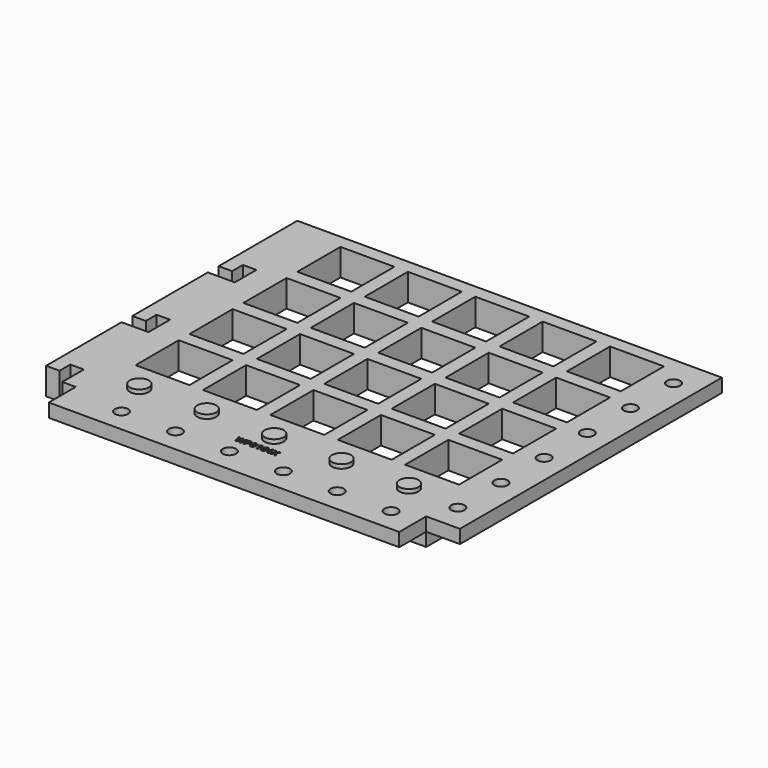
from build123d import *

# Parameters (mm, degrees)
F0_W          = 260
F0_H          = 210
F0_W_2        = 40
F0_H_2        = 40
F1_DEPTH      = 20
F2_DEPTH      = 33
F3_W          = 260
F3_H          = 10
F4_DEPTH      = 25
F5_R          = 4.95
F6_DEPTH      = 25
F7_W          = 243
F7_H          = 10
F8_DEPTH      = 25
F9_R          = 4.95
F10_DEPTH     = 25
F11_W         = 243
F11_H         = 20
F12_DEPTH     = 30
F14_DEPTH     = 25
F15_R         = 7.05
F16_DEPTH     = 3
F17_TEXT_SIZE = 6.9444444444
F18_DEPTH     = 3


# Not quite as in the source:
# - Text() gives the source's letters only with a copy of the font that has no kerning and outlines rounded to 1/6400 em; it was checked with that copy


with BuildPart() as f1:
    # F0 (on Top) → F1 (new body)
    with BuildSketch(Plane.XY):
        Rectangle(F0_W, F0_H)
        with Locations((-100, -75)):
            Rectangle(F0_W_2, F0_H_2, mode=Mode.SUBTRACT)
        with Locations((-50, -75)):
            Rectangle(F0_W_2, F0_H_2, mode=Mode.SUBTRACT)
        with Locations((-100, -25)):
            Rectangle(F0_W_2, F0_H_2, mode=Mode.SUBTRACT)
        with Locations((-50, -25)):
            Rectangle(F0_W_2, F0_H_2, mode=Mode.SUBTRACT)
        with Locations((0, -75)):
            Rectangle(F0_W_2, F0_H_2, mode=Mode.SUBTRACT)
        with Locations((50, -75)):
            Rectangle(F0_W_2, F0_H_2, mode=Mode.SUBTRACT)
        with Locations((100, -75)):
            Rectangle(F0_W_2, F0_H_2, mode=Mode.SUBTRACT)
        with Locations((0, -25)):
            Rectangle(F0_W_2, F0_H_2, mode=Mode.SUBTRACT)
        with Locations((50, -25)):
            Rectangle(F0_W_2, F0_H_2, mode=Mode.SUBTRACT)
        with Locations((100, -25)):
            Rectangle(F0_W_2, F0_H_2, mode=Mode.SUBTRACT)
        with Locations((-100, 25)):
            Rectangle(F0_W_2, F0_H_2, mode=Mode.SUBTRACT)
        with Locations((-50, 25)):
            Rectangle(F0_W_2, F0_H_2, mode=Mode.SUBTRACT)
        with Locations((-100, 75)):
            Rectangle(F0_W_2, F0_H_2, mode=Mode.SUBTRACT)
        with Locations((-50, 75)):
            Rectangle(F0_W_2, F0_H_2, mode=Mode.SUBTRACT)
        with Locations((0, 25)):
            Rectangle(F0_W_2, F0_H_2, mode=Mode.SUBTRACT)
        with Locations((50, 25)):
            Rectangle(F0_W_2, F0_H_2, mode=Mode.SUBTRACT)
        with Locations((100, 25)):
            Rectangle(F0_W_2, F0_H_2, mode=Mode.SUBTRACT)
        with Locations((0, 75)):
            Rectangle(F0_W_2, F0_H_2, mode=Mode.SUBTRACT)
        with Locations((50, 75)):
            Rectangle(F0_W_2, F0_H_2, mode=Mode.SUBTRACT)
        with Locations((100, 75)):
            Rectangle(F0_W_2, F0_H_2, mode=Mode.SUBTRACT)
    extrude(amount=F1_DEPTH)

    # F2 (add): a face of the model
    f2_faces = [f1.faces().sort_by_distance(p)[0] for p in [
        (0, -105, 10),
    ]]
    extrude(f2_faces, amount=F2_DEPTH)

    # F3 (on face) → F4 (join)
    with BuildSketch(Plane.XZ.offset(138)):
        with Locations((0, 15)):
            Rectangle(F3_W, F3_H)
    extrude(amount=F4_DEPTH)

    # F5 (on face) → F6 (cut)
    with BuildSketch(Plane.XY.offset(20)):
        with Locations((110, -145.5)):
            Circle(F5_R)
        with Locations((70, -145.5)):
            Circle(F5_R)
        with Locations((30, -145.5)):
            Circle(F5_R)
        with Locations((-10, -145.5)):
            Circle(F5_R)
        with Locations((-50, -145.5)):
            Circle(F5_R)
        with Locations((-90, -145.5)):
            Circle(F5_R)
    extrude(amount=-F6_DEPTH, mode=Mode.SUBTRACT)

    # F7 (on face) → F8 (join)
    with BuildSketch(Plane.YZ.offset(130)):
        with Locations((-16.5, 15)):
            Rectangle(F7_W, F7_H)
    extrude(amount=F8_DEPTH)

    # F9 (on face) → F10 (cut)
    with BuildSketch(Plane.XY.offset(20)):
        with Locations((137.5, -118)):
            Circle(F9_R)
        with Locations((137.5, -78)):
            Circle(F9_R)
        with Locations((137.5, -38)):
            Circle(F9_R)
        with Locations((137.5, 2)):
            Circle(F9_R)
        with Locations((137.5, 42)):
            Circle(F9_R)
        with Locations((137.5, 82)):
            Circle(F9_R)
    extrude(amount=-F10_DEPTH, mode=Mode.SUBTRACT)

    # F11 (on face) → F12 (join)
    with BuildSketch(Plane(origin=(-130, 0, 0), x_dir=(0, -1, 0), z_dir=(-1, 0, 0))):
        with Locations((16.5, 10)):
            Rectangle(F11_W, F11_H)
    extrude(amount=F12_DEPTH)

    # F13 (on face) → F14 (cut)
    with BuildSketch(Plane.XY.offset(20)):
        Polygon((-160, -128), (-160, -138), (-140, -138), (-140, -118), (-150, -118), (-150, -128), align=None)
        Polygon((-140, -58), (-140, -38), (-150, -38), (-150, -48), (-160, -48), (-160, -58), align=None)
        Polygon((-140, 22), (-140, 42), (-150, 42), (-150, 32), (-160, 32), (-160, 22), align=None)
    extrude(amount=-F14_DEPTH, mode=Mode.SUBTRACT)

    # F15 (on face) → F16 (join)
    with BuildSketch(Plane.XY.offset(20)):
        with Locations((100, -116.5)):
            Circle(F15_R)
        with Locations((50, -116.5)):
            Circle(F15_R)
        with Locations((0, -116.5)):
            Circle(F15_R)
        with Locations((-50, -116.5)):
            Circle(F15_R)
        with Locations((-100, -116.5)):
            Circle(F15_R)
    extrude(amount=F16_DEPTH)

    # F17 (on face) → F18 (cut)
    with BuildSketch(Plane.XY.offset(20)):
        with Locations((-17.0128038194, -133)):
            Text('WP0164X', F17_TEXT_SIZE, font='Open Sans', font_style=FontStyle.BOLD, text_align=(TextAlign.LEFT, TextAlign.BOTTOM))
    extrude(amount=-F18_DEPTH, mode=Mode.SUBTRACT)


solid = f1.part
